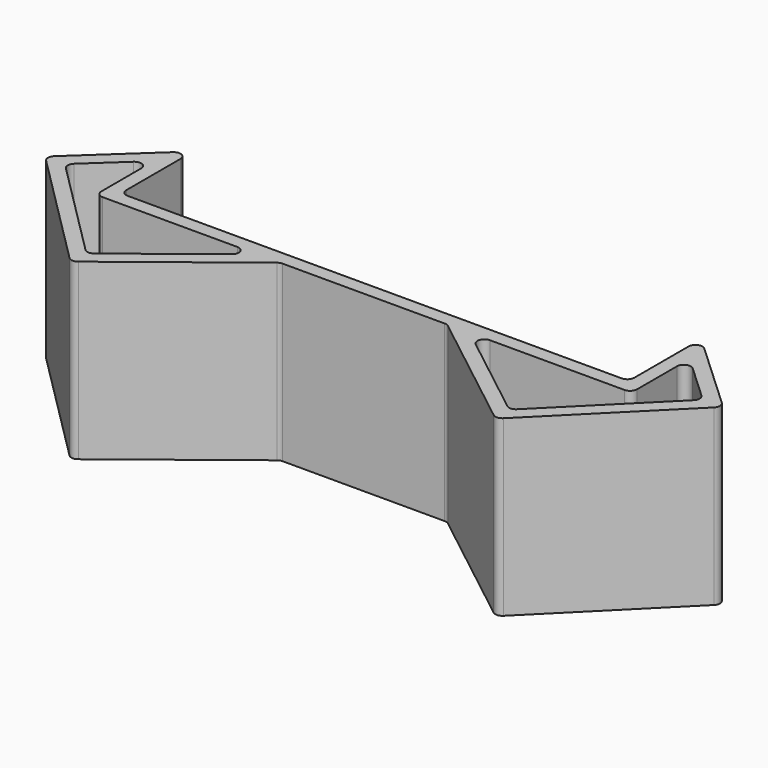
from build123d import *

# Parameters (mm, degrees)
F1_DEPTH = 25
F2_R     = 1


# Not quite as in the source:
# - a feature names something its author has since deleted; it is built from what else it names


with BuildPart() as f1:
    # F0 (on Top) → F1 (new body)
    with BuildSketch(Plane.XY):
        Polygon((0, -2), (0, 0), (-36.5, 0), (-36.5, 10.3007538181), (-38.5, 8.4454781792), (-38.5, -2), (-15.248538491, -2), (-12, -2), align=None)
        Polygon((36.5, 0), (0, 0), (0, -2), (12, -2), (15.248538491, -2), (38.5, -2), (38.5, 8.4454781792), (36.5, 10.3007538181), align=None)
        Polygon((-38.5, 8.4454781792), (-36.5, 10.3007538181), (-36.5, 13.0287654926), (-38.5, 11.1734898537), align=None)
        Polygon((-30.5484807652, -16.4916614154), (-12, -2), (-15.248538491, -2), (-30.3854576709, -13.8262573849), (-45.844322202, 1.6326071462), (-47.3116243561, 0.2714821755), align=None)
        Polygon((15.248538491, -2), (12, -2), (30.5484807652, -16.4916614154), (47.3116243561, 0.2714821755), (45.844322202, 1.6326071462), (30.3854576709, -13.8262573849), align=None)
        Polygon((36.5, 13.0287654926), (36.5, 10.3007538181), (38.5, 8.4454781792), (38.5, 11.1734898537), align=None)
        Polygon((-45.844322202, 1.6326071462), (-38.5, 8.4454781792), (-38.5, 11.1734898537), (-47.259531868, 3.0478168121), align=None)
        Polygon((38.5, 11.1734898537), (38.5, 8.4454781792), (45.844322202, 1.6326071462), (47.259531868, 3.0478168121), align=None)
        Polygon((-47.3116243561, 0.2714821755), (-45.844322202, 1.6326071462), (-47.259531868, 3.0478168121), (-48.726834022, 1.6866918414), align=None)
        Polygon((45.844322202, 1.6326071462), (47.3116243561, 0.2714821755), (48.726834022, 1.6866918414), (47.259531868, 3.0478168121), align=None)
    extrude(amount=F1_DEPTH)

    # F2
    f2_edges = [f1.edges().sort_by_distance(p)[0] for p in [
        (-36.5, 0, 12.5),
        (-38.5, -2, 12.5),
        (-15.248538, -2, 12.5),
        (15.248538, -2, 12.5),
        (30.385458, -13.826257, 12.5),
        (38.5, -2, 12.5),
        (38.5, 8.445478, 12.5),
        (45.844322, 1.632607, 12.5),
        (12, -2, 12.5),
        (30.548481, -16.491661, 12.5),
        (36.5, 13.028765, 12.5),
        (36.5, 0, 12.5),
        (48.726834, 1.686692, 12.5),
        (-45.844322, 1.632607, 12.5),
        (-48.726834, 1.686692, 12.5),
        (-36.5, 13.028765, 12.5),
        (-30.548481, -16.491661, 12.5),
        (-12, -2, 12.5),
        (-30.385458, -13.826257, 12.5),
        (-38.5, 8.445478, 12.5),
    ]]
    fillet(f2_edges, radius=F2_R)


solid = f1.part
